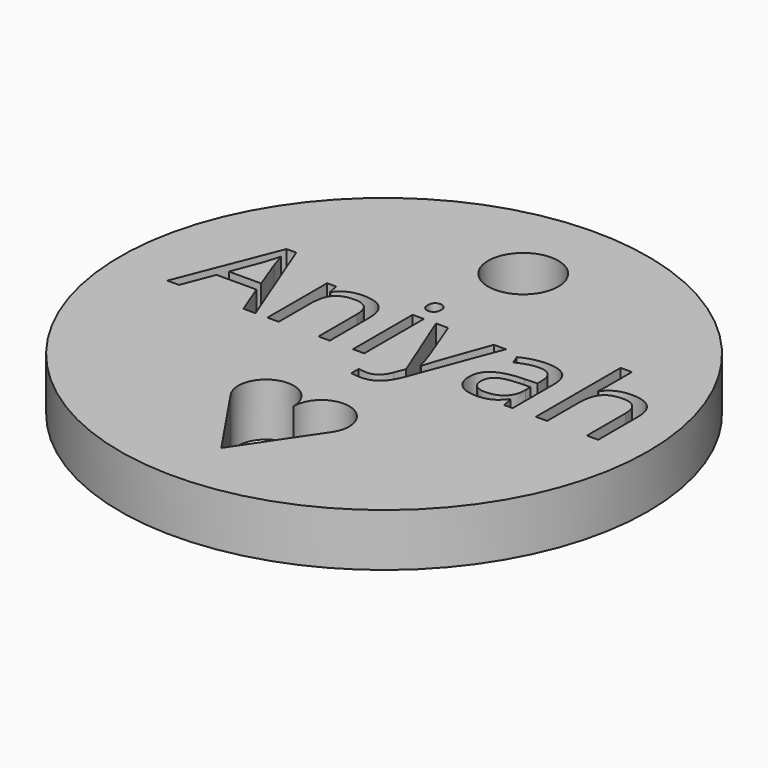
from build123d import *

# Parameters (mm, degrees)
F0_R         = 19.05
F1_DEPTH     = 3.81
F2_TEXT_SIZE = 10.0549260231
F3_DEPTH     = 4
F4_R         = 2.5323932176
F5_DEPTH     = 25.4
F7_DEPTH     = 25.4


# Not quite as in the source:
# - Text() gives the source's letters only with a copy of the font that has no kerning and outlines rounded to 1/6400 em; it was checked with that copy


with BuildPart() as f1:
    # F0 (on Top) → F1 (new body)
    with BuildSketch(Plane.XY):
        Circle(F0_R)
    extrude(amount=F1_DEPTH)

    # F2 (on Top) → F3 (cut)
    with BuildSketch(Plane.XY):
        with Locations((-15.1335613158, -0.6398935713)):
            Text('Aniyah', F2_TEXT_SIZE, font='Open Sans', text_align=(TextAlign.LEFT, TextAlign.BOTTOM))
    extrude(amount=F3_DEPTH, mode=Mode.SUBTRACT)

    # F4 (on Top) → F5 (cut)
    with BuildSketch(Plane.XY):
        with Locations((0, 12.553293258)):
            Circle(F4_R)
    extrude(amount=F5_DEPTH, mode=Mode.SUBTRACT)

    # F6 (on Top) → F7 (cut)
    with BuildSketch(Plane.XY):
        with BuildLine():
            ThreePointArc((-3.6573010907, -9.269532534), (-1.4145950895, -10.0624071457), (0, -8.15))
            ThreePointArc((0, -8.15), (-2.5854049105, -6.2375928543), (-3.6573010907, -9.269532534))
        make_face()
        with BuildLine():
            Line((0, -14.6836218104), (0, -8.15))
            ThreePointArc((0, -8.15), (-1.4145950895, -10.0624071457), (-3.6573010907, -9.269532534))
            Line((-3.6573010907, -9.269532534), (0, -14.6836218104))
        make_face()
        with BuildLine():
            ThreePointArc((3.6573010907, -9.269532534), (1.4145950895, -10.0624071457), (0, -8.15))
            Line((0, -8.15), (0, -14.6836218104))
            Line((0, -14.6836218104), (3.6573010907, -9.269532534))
        make_face()
        with BuildLine():
            ThreePointArc((4, -8.15), (2, -6.15), (0, -8.15))
            ThreePointArc((0, -8.15), (1.4145950895, -10.0624071457), (3.6573010907, -9.269532534))
            ThreePointArc((3.6573010907, -9.269532534), (3.9124071457, -8.7354049105), (4, -8.15))
        make_face()
    extrude(amount=F7_DEPTH, mode=Mode.SUBTRACT)


solid = f1.part
